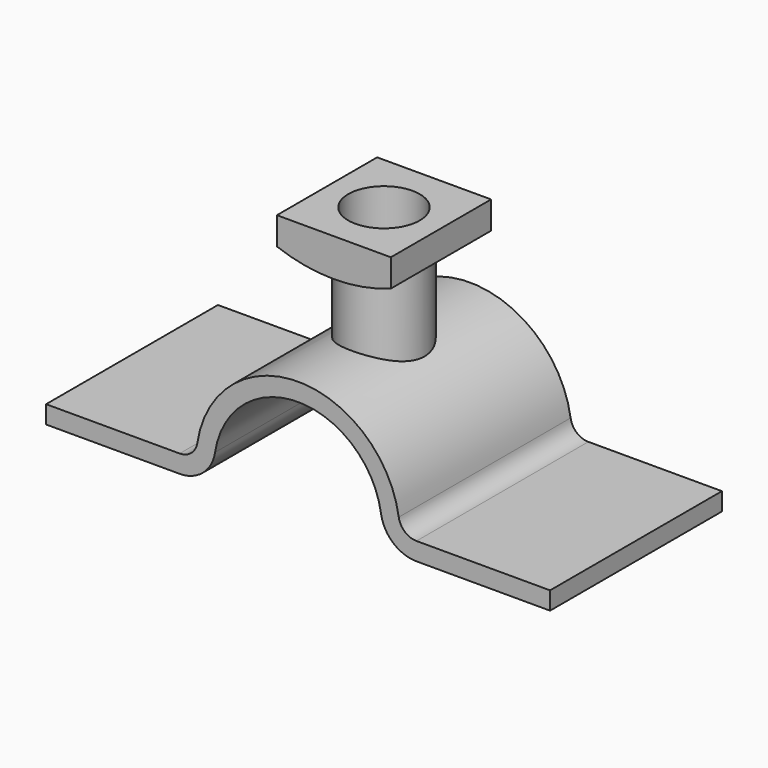
from build123d import *

# Parameters (mm, degrees)
F1_DEPTH = 38.1
F3_DEPTH = 22.225
F4_R     = 14.351
F5_REACH = 121.9987572146
F6_R     = 12.6746
F7_DEPTH = 81.4079995473


# Not quite as in the source:
# - a feature names something its author has since deleted; it is built from what else it names


with BuildPart() as f1:
    # F0 (on Front) → F1 (new body, symmetric)
    with BuildSketch(Plane.XZ):
        with BuildLine():
            ThreePointArc((41.9913857052, 0), (37.8505272155, 1.5358758877), (35.7127694215, 5.4005382775))
            ThreePointArc((35.7127694215, 5.4005382775), (0, 36.1188), (-35.7127694215, 5.4005382775))
            ThreePointArc((-35.7127694215, 5.4005382775), (-37.8505272155, 1.5358758877), (-41.9913857052, 0))
            Line((-41.9913857052, 0), (-89.3826, 0))
            Line((-89.3826, 0), (-89.3826, -6.3499995473))
            Line((-89.3826, -6.3499995473), (-41.9913857052, -6.3499995473))
            ThreePointArc((-41.9913857052, -6.3499995473), (-33.7096690211, -3.2782478815), (-29.4341535854, 4.4510766227))
            ThreePointArc((-29.4341535854, 4.4510766227), (0, 29.7688004527), (29.4341535854, 4.4510766227))
            ThreePointArc((29.4341535854, 4.4510766227), (33.7096690211, -3.2782478815), (41.9913857052, -6.3499995473))
            Line((41.9913857052, -6.3499995473), (89.3826, -6.3499995473))
            Line((89.3826, -6.3499995473), (89.3826, 0))
            Line((89.3826, 0), (41.9913857052, 0))
        make_face()
    extrude(amount=F1_DEPTH, both=True)



with BuildPart() as f3:
    # F2 (on Front) → F3 (new body, symmetric)
    with BuildSketch(Plane.XZ):
        with BuildLine():
            Line((20.2057, 75.057), (0, 75.057))
            Line((0, 75.057), (-20.2057, 75.057))
            Line((-20.2057, 75.057), (-20.2057, 65.278))
            ThreePointArc((-20.2057, 65.278), (0, 61.6607352251), (20.2057, 65.278))
            Line((20.2057, 65.278), (20.2057, 75.057))
        make_face()
    extrude(amount=F3_DEPTH, both=True)


with BuildPart() as f1_1:
    add(f1.part)

    add(f3.part)  # F5 merges F3
    f5_end = f1_1.faces().sort_by_distance((0, 0, 36.1188))[0]
    # F4 (on face) → F5 (join, up to a face of the model that its end follows)
    with BuildSketch(Plane.XY.offset(75.057)):
        Circle(F4_R)
    f5_long = extrude(amount=-F5_REACH, mode=Mode.PRIVATE)
    add(split(f5_long, bisect_by=f5_end, keep=Keep.TOP, mode=Mode.PRIVATE))

    # F6 (on face) → F7 (cut, through all)
    with BuildSketch(Plane.XY.offset(75.057)):
        Circle(F6_R)
    extrude(amount=-F7_DEPTH, mode=Mode.SUBTRACT)


solid = f1_1.part
